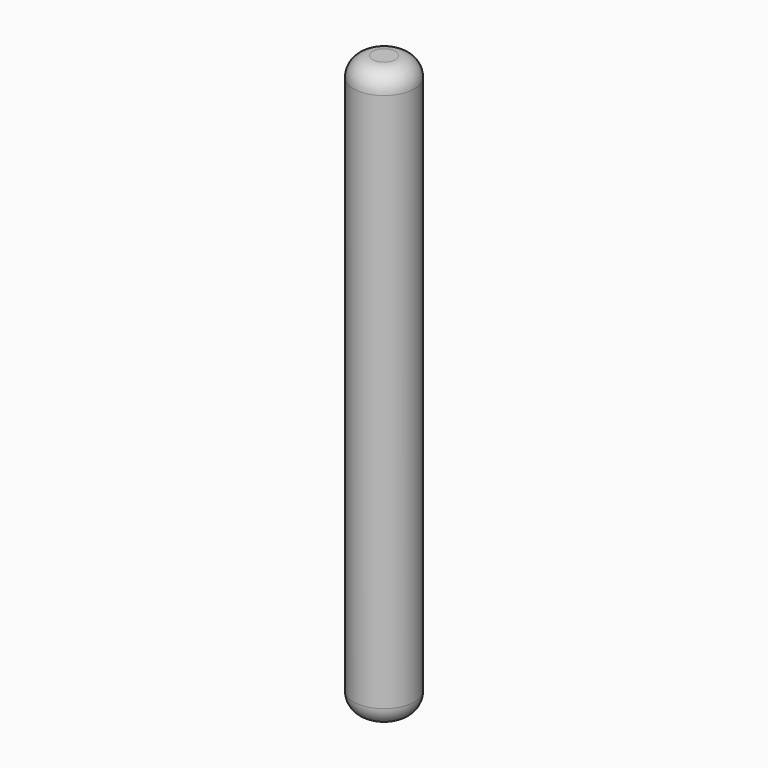
from build123d import *

# Parameters (mm, degrees)
F1_R     = 1.5875
F2_DEPTH = 30
F3_R     = 1


with BuildPart() as f2:
    # F1 (on Top) → F2 (new body)
    with BuildSketch(Plane.XY):
        Circle(F1_R)
    extrude(amount=F2_DEPTH)

    # F3
    f3_edges = [f2.edges().sort_by_distance(p)[0] for p in [
        (-1.5875, 0, 30),
        (-1.5875, 0, 0),
    ]]
    fillet(f3_edges, radius=F3_R)


solid = f2.part
